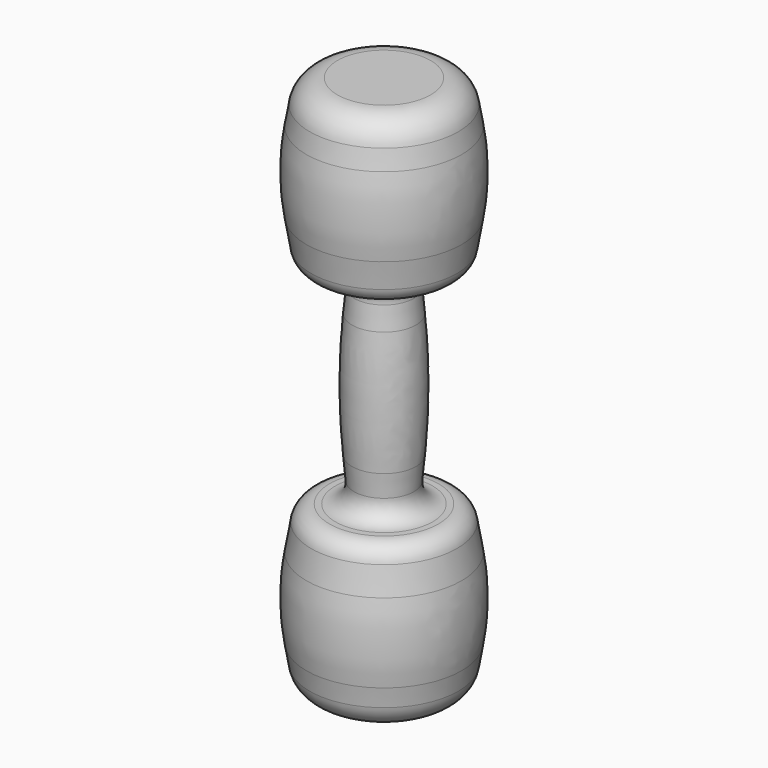
from build123d import *

# Parameters (mm, degrees)
F2_R = 4
F3_R = 50
F4_R = 6
F5_R = 150


with BuildPart() as f1:
    # F0 (on Front) → F1 (revolve)
    with BuildSketch(Plane.XZ):
        Polygon((15, 57.5), (0, 57.5), (0, 56), (13.5, 56), (16.2428571429, 40), (13.5, 24), (4.5, 24), (0.6066159112, 24), (0.6066159112, 22.5), (4.6333333333, 22.5), (6.6333333333, 0), (4.6333333333, -22.5), (0.3456167178, -22.5), (0.3456167178, -24), (4.5, -24), (13.5, -24), (16.5019892156, -40.1757322252), (13.5, -56), (0, -56), (0, -57.5), (15, -57.5), (18, -40), (15, -22.5), (6, -22.5), (8, 0), (6, 22.5), (15, 22.5), (18, 40), align=None)
    revolve(axis=Axis((0, 0, 66.6587725282), (0, 0, -1)))

    # F2
    f2_edges = [f1.edges().sort_by_distance(p)[0] for p in [
        (-15, 0, -22.5),
        (-6, 0, -22.5),
        (-6, 0, 22.5),
        (-15, 0, 22.5),
    ]]
    fillet(f2_edges, radius=F2_R)

    # F3
    f3_edges = [f1.edges().sort_by_distance(p)[0] for p in [
        (-18, 0, 40),
        (-18, 0, -40),
    ]]
    fillet(f3_edges, radius=F3_R)

    # F4
    f4_edges = [f1.edges().sort_by_distance(p)[0] for p in [
        (-15, 0, 57.5),
        (-15, 0, -57.5),
    ]]
    fillet(f4_edges, radius=F4_R)

    # F5
    f5_edges = [f1.edges().sort_by_distance(p)[0] for p in [
        (-8, 0, 0),
    ]]
    fillet(f5_edges, radius=F5_R)


solid = f1.part
